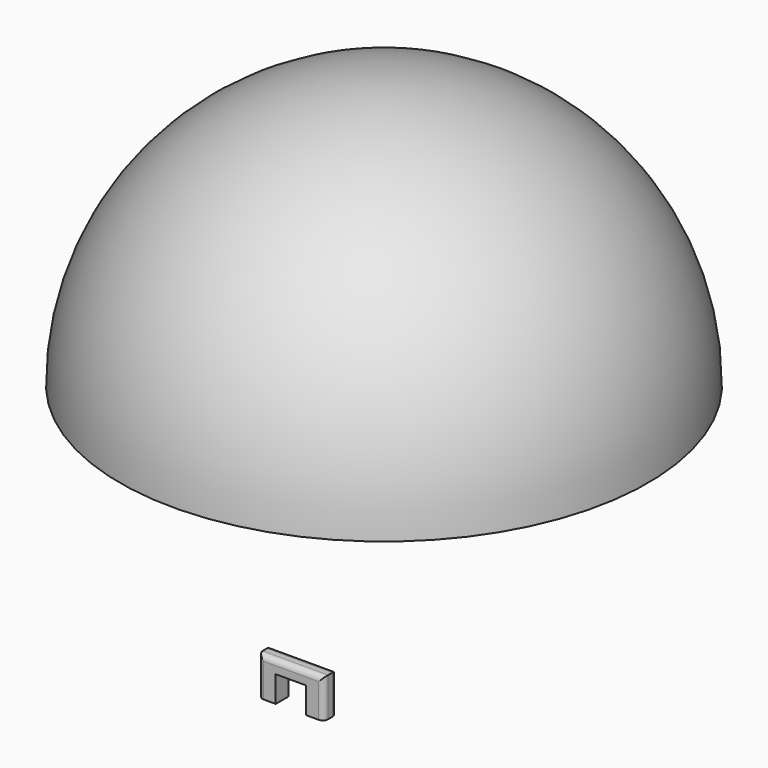
from build123d import *

# Parameters (mm, degrees)
F2_T     = -0.127
F5_T     = -0.127
F9_DEPTH = 1.905
F10_R    = 0.635


# Not quite as in the source:
# - the program builds the solid bodies; features that only make, move or delete a surface that nothing else refers to are left out


with BuildPart() as f1:
    # F0 (on Front) → F1 (revolve)
    with BuildSketch(Plane.XZ):
        with BuildLine():
            Line((0, 0), (0, 31.419273907))
            ThreePointArc((0, 31.419273907), (-22.2167816396, 22.2167816396), (-31.419273907, 0))
            Line((-31.419273907, 0), (0, 0))
        make_face()
    revolve(axis=Axis((0, 0, 0), (0, 0, -1)))

    # F2
    f2_openings = [f1.faces().sort_by_distance(p)[0] for p in [
        (0, 0, 0),
    ]]
    offset(amount=F2_T, openings=f2_openings)


with BuildPart() as f4:
    # F3 (on Front) → F4 (revolve)
    with BuildSketch(Plane.XZ):
        with BuildLine():
            Line((0, 0), (10.8270294, 0))
            ThreePointArc((10.8270294, 0), (7.6558659088, 7.6558659088), (0, 10.8270294))
            Line((0, 10.8270294), (0, 0))
        make_face()
    revolve(axis=Axis((0, 0, 5.4135147), (0, 0, 1)))

    # F5
    f5_openings = [f4.faces().sort_by_distance(p)[0] for p in [
        (0, 0, 0),
    ]]
    offset(amount=F5_T, openings=f5_openings)


with BuildPart() as f9:
    # F8 (on Front) → F9 (new body)
    with BuildSketch(Plane.XZ):
        Polygon((-13.4343560785, -31.6628441215), (-13.4343560785, -36.2952388823), (-11.370417662, -36.2952388823), (-11.370417662, -33.1763960421), (-7.7470592223, -33.1763960421), (-7.7470592223, -36.2952388823), (-5.6372559629, -36.2952388823), (-5.6372559629, -31.6628441215), align=None)
    extrude(amount=F9_DEPTH)

    # F10
    f10_edges = [f9.edges().sort_by_distance(p)[0] for p in [
        (-9.535806, -1.905, -31.662844),
        (-9.535806, 0, -31.662844),
        (-5.637256, -1.905, -33.979042),
        (-5.637256, 0, -33.979042),
        (-13.434356, 0, -33.979042),
        (-13.434356, -1.905, -33.979042),
    ]]
    fillet(f10_edges, radius=F10_R)


solid = Compound([f1.part, f4.part, f9.part])
